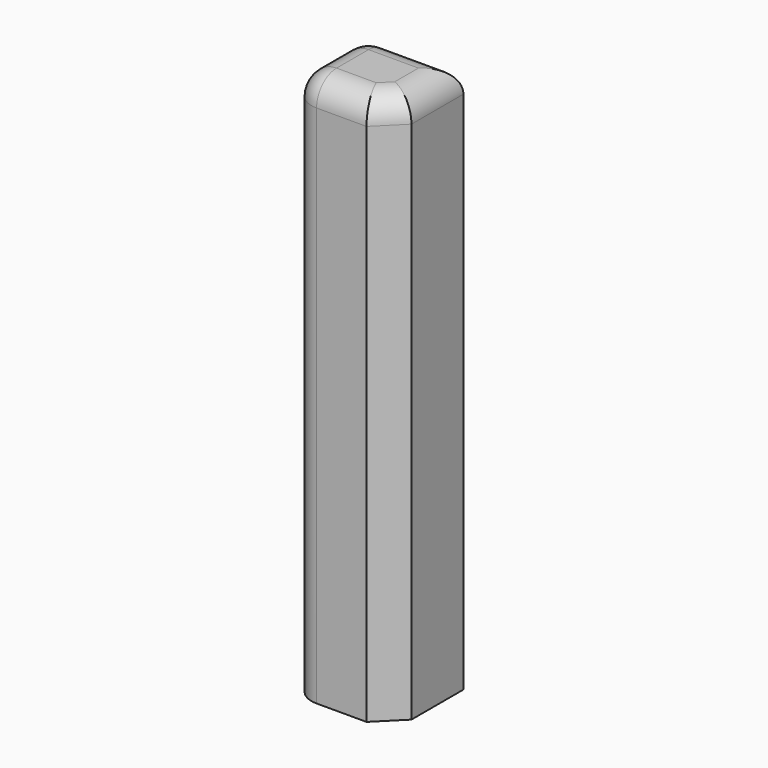
from build123d import *

# Parameters (mm, degrees)
F0_W     = 20
F0_H     = 100
F1_DEPTH = 10
F2_W     = 20
F2_H     = 100
F2_R     = 3
F3_DEPTH = 8
F4_SIZE  = 5
F5_R     = 5
F6_DEPTH = 10
F7_R     = 5


with BuildPart() as f1:
    # F0 (on Front) → F1 (new body)
    with BuildSketch(Plane.XZ):
        with Locations((0, 40)):
            Rectangle(F0_W, F0_H)
    extrude(amount=F1_DEPTH)

    # F2 (on face) → F3 (join)
    with BuildSketch(Plane(origin=(0, 0, 0), x_dir=(-1, 0, 0), z_dir=(0, 1, 0))):
        with Locations((0, 40)):
            Rectangle(F2_W, F2_H)
        Circle(F2_R, mode=Mode.SUBTRACT)
    extrude(amount=F3_DEPTH)

    # F4
    f4_edges = [f1.edges().sort_by_distance(p)[0] for p in [
        (10, -10, 40),
    ]]
    chamfer(f4_edges, length=F4_SIZE)

    # F5
    f5_edges = [f1.edges().sort_by_distance(p)[0] for p in [
        (-10, -10, 40),
        (-10, 8, 40),
    ]]
    fillet(f5_edges, radius=F5_R)

    # F6 (add): a face of the model
    f6_faces = [f1.faces().sort_by_distance(p)[0] for p in [
        (-0.0262777066, -0.7278062427, 90),
    ]]
    extrude(f6_faces, amount=F6_DEPTH)

    # F7
    f7_edges = [f1.edges().sort_by_distance(p)[0] for p in [
        (10, 1.5, 100),
        (2.5, 8, 100),
        (-10, -1, 100),
        (7.5, -7.5, 100),
        (-8.535534, -8.535534, 100),
        (0, -10, 100),
        (-8.535534, 6.535534, 100),
    ]]
    fillet(f7_edges, radius=F7_R)


solid = f1.part
